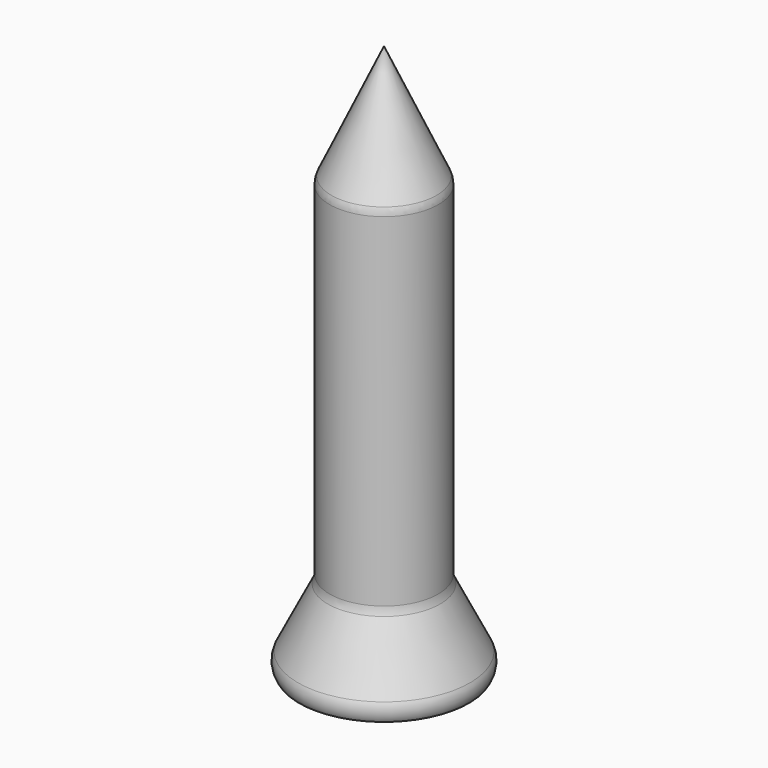
from build123d import *

# Parameters (mm, degrees)
F3_T = -2.54
F4_R = 5.08


# Not quite as in the source:
# - a fillet or chamfer that OpenCascade refuses, or shapes differently, is made with other operations: its cross-section is extruded or revolved along the edge and cut away or added


with BuildPart() as f2:
    # F0 (on Right) → F2 (revolve)
    with BuildSketch(Plane.YZ):
        Polygon((0, -77.1136805415), (0, 0), (0, 75.9008899331), (-15.0823583826, 43.1482791901), (-15.0823583826, -54.3898443918), (-26.3941269368, -77.1136805415), align=None)
    revolve(axis=Axis((0, 0, 37.9504449666), (0, 0, 1)))

    # F3
    f3_openings = [f2.faces().sort_by_distance(p)[0] for p in [
        (0, 0, -77.113681),
    ]]
    offset(amount=F3_T, openings=f3_openings, kind=Kind.INTERSECTION)

    # F4
    f4_edges = [f2.edges().sort_by_distance(p)[0] for p in [
        (0, 15.082358, 43.148279),
        (0, 15.082358, -54.389844),
        (0, -15.082358, -5.620783),
    ]]
    fillet(f4_edges, radius=F4_R)

    # F5: fillet of radius 5.08 on 3 edges, made by hand

    # F5_s1 → F5_t2 (revolve, cut)
    with BuildSketch(Plane.YZ):
        with BuildLine():
            ThreePointArc((-23.8701527835, -72.0433526939), (-24.3927830464, -74.6204948412), (-23.5568230573, -77.1136805415))
            Line((-23.5568230573, -77.1136805415), (-26.3941269368, -77.1136805415))
            Line((-26.3941269368, -77.1136805415), (-23.8701527835, -72.0433526939))
        make_face()
    revolve(axis=Axis((0, 0, -77.1136805415), (0, 0, 1)), mode=Mode.SUBTRACT)


solid = f2.part
